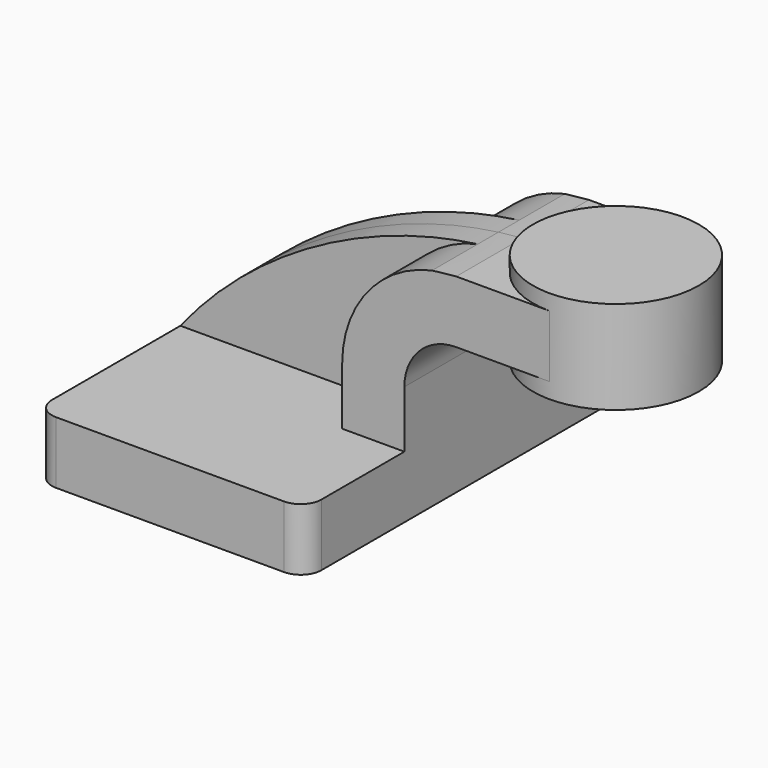
from build123d import *

# Parameters (mm, degrees)
F1_DEPTH = 63.5
F0_W     = 25.4
F0_H     = 19.05
F2_DEPTH = 25.4
F3_DEPTH = 7.9375
F5_R     = 6.35


# Not quite as in the source:
# - a feature names something its author has since deleted; it is built from what else it names


with BuildPart() as f1:
    # F0 (on Front) → F1 (new body, symmetric)
    with BuildSketch(Plane.XZ):
        Polygon((41.275, -9.525), (41.275, 9.525), (22.225, 9.525), (-41.275, 9.525), (-41.275, -9.525), align=None)
    extrude(amount=F1_DEPTH, both=True)

    # F0 (on Front) → F2 (join, symmetric)
    with BuildSketch(Plane.XZ):
        with BuildLine():
            Line((22.225, 9.525), (41.275, 9.525))
            Line((41.275, 9.525), (41.275, 27.0002))
            ThreePointArc((41.275, 27.0002), (45.9246798487, 38.2255201513), (57.15, 42.8752))
            Line((57.15, 42.8752), (60.325, 42.8752))
            Line((60.325, 42.8752), (60.325, 61.9252))
            Line((60.325, 61.9252), (57.15, 61.9252))
            add(Edge.make_bspline(
                [(49.7646190409, 61.1353984481), (52.2104568014, 61.4669327128), (54.6731104701, 61.7311893911), (57.15, 61.9252)],
                knots=[104.645371818, 104.645371818, 104.645371818, 104.645371818, 111.5045361635, 111.5045361635, 111.5045361635, 111.5045361635], degree=3))
            ThreePointArc((49.7646190409, 61.1353984481), (29.9682960891, 48.9298739032), (22.225, 27.0002))
            Line((22.225, 27.0002), (22.225, 9.525))
        make_face()
        with Locations((73.025, 52.4002)):
            Rectangle(F0_W, F0_H)
    extrude(amount=F2_DEPTH, both=True)

    # F0 (on Front) → F3 (join, symmetric)
    with BuildSketch(Plane.XZ):
        with BuildLine():
            Line((-41.275, 9.525), (22.225, 9.525))
            Line((22.225, 9.525), (22.225, 27.0002))
            ThreePointArc((22.225, 27.0002), (29.9682960891, 48.9298739032), (49.7646190409, 61.1353984481))
            add(Edge.make_bspline(
                [(-41.275, 9.525), (-20.9502066659, 35.3602907495), (12.4502190704, 56.0774169419), (49.7646190409, 61.1353984481)],
                knots=[0, 0, 0, 0, 104.645371818, 104.645371818, 104.645371818, 104.645371818], degree=3))
        make_face()
    extrude(amount=F3_DEPTH, both=True)

    # F0 (on Front) → F4 (revolve)
    with BuildSketch(Plane.XZ):
        Polygon((85.725, 61.9252), (85.725, 42.8752), (85.725, 38.1), (111.125, 38.1), (111.125, 66.675), (85.725, 66.675), align=None)
    revolve(axis=Axis((85.725, 0, 52.3875), (0, 0, 1)))

    # F5
    f5_edges = [f1.edges().sort_by_distance(p)[0] for p in [
        (41.275, -63.5, 0),
        (41.275, 63.5, 0),
        (-41.275, 63.5, 0),
        (-41.275, -63.5, 0),
    ]]
    fillet(f5_edges, radius=F5_R)


solid = f1.part
